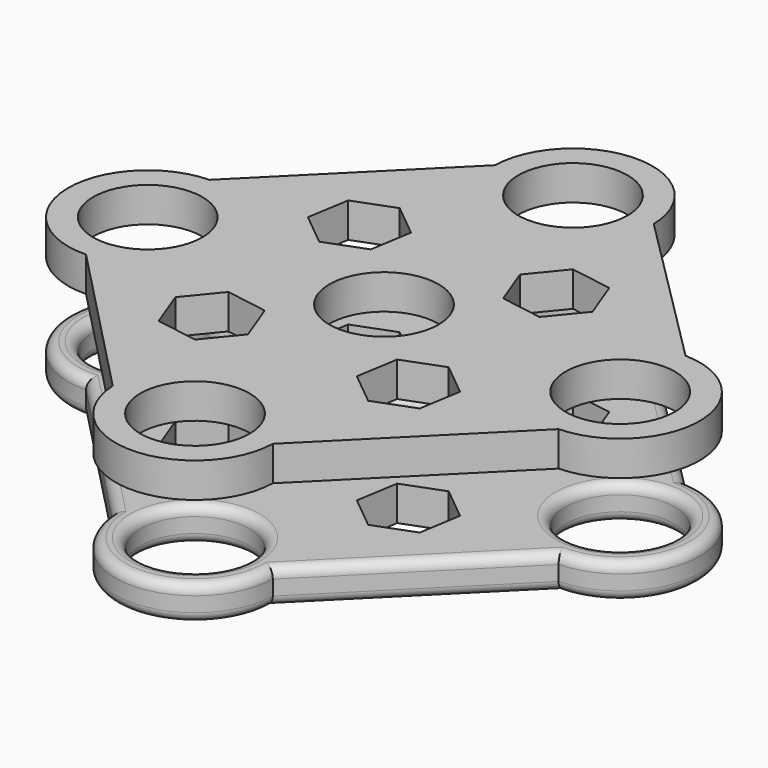
from build123d import *

# Parameters (mm, degrees)
F0_R     = 11
F1_DEPTH = 7
F3_R     = 2
F4_R     = 1.99999


# Not quite as in the source:
# - a fillet or chamfer is up to 0.001 mm smaller than in the source, because OpenCascade refuses the exact size


with BuildPart() as f1:
    # F0 (on Top) → F1 (new body)
    with BuildSketch(Plane.XY):
        with BuildLine():
            Line((-15.9957736565, 47.9499164564), (-47.9659518715, 15.9953969734))
            ThreePointArc((-47.9659518715, 15.9953969734), (-63.5777739911, -0.3757513624), (-47.2144492409, -15.9957734767))
            Line((-47.2144492409, -15.9957734767), (-15.9838429391, -48.3010503735))
            ThreePointArc((-15.9838429391, -48.3010503735), (0.1596400242, -63.5813903344), (15.9950047504, -47.9819654893))
            Line((15.9950047504, -47.9819654893), (47.9819799, -15.9950043902))
            ThreePointArc((47.9819799, -15.9950043902), (63.5821787222, 0.0160362946), (47.9499165377, 15.9957736546))
            Line((47.9499165377, 15.9957736546), (15.9961341611, 47.9338853509))
            ThreePointArc((15.9961341611, 47.9338853509), (0.0080175792, 63.5821847497), (-15.9957736565, 47.9499164564))
        make_face()
        with Locations((0, -47.5821867585)):
            Circle(F0_R, mode=Mode.SUBTRACT)
        with Locations((-47.5821867585, 0)):
            Circle(F0_R, mode=Mode.SUBTRACT)
        Polygon((-24.1507935557, -26.5329984332), (-27.1666148322, -18.5563192395), (-21.7665186508, -11.9562018039), (-13.350601193, -13.3327635621), (-10.3347799165, -21.3094427558), (-15.7348760979, -27.9095601914), align=None, mode=Mode.SUBTRACT)
        Circle(F0_R, mode=Mode.SUBTRACT)
        Polygon((27.9095601914, -15.7348760979), (26.5329984332, -24.1507935557), (18.5563192395, -27.1666148322), (11.9562018039, -21.7665186508), (13.3327635621, -13.350601193), (21.3094427558, -10.3347799165), align=None, mode=Mode.SUBTRACT)
        with Locations((47.5821867585, 0)):
            Circle(F0_R, mode=Mode.SUBTRACT)
        Polygon((-27.9095601914, 15.7348760979), (-26.5329984332, 24.1507935557), (-18.5563192395, 27.1666148322), (-11.9562018039, 21.7665186508), (-13.3327635621, 13.350601193), (-21.3094427558, 10.3347799165), align=None, mode=Mode.SUBTRACT)
        with Locations((0, 47.5821867585)):
            Circle(F0_R, mode=Mode.SUBTRACT)
        Polygon((15.7348760979, 27.9095601914), (24.1507935557, 26.5329984332), (27.1666148322, 18.5563192395), (21.7665186508, 11.9562018039), (13.350601193, 13.3327635621), (10.3347799165, 21.3094427558), align=None, mode=Mode.SUBTRACT)
    extrude(amount=F1_DEPTH)


with BuildPart() as f2_1:
    # F2: copy of F1
    add(f1.part.moved(Location((0, 0, 22))))


with BuildPart() as f1_1:
    add(f1.part)

    # F3
    f3_edges = [f1_1.edges().sort_by_distance(p)[0] for p in [
        (-31.980863, 31.972657, 7),
    ]]
    fillet(f3_edges, radius=F3_R)

    # F4 (radius 2 in the source; OpenCascade refuses exactly that, so slightly less here)
    f4_edges = [f1_1.edges().sort_by_distance(p)[0] for p in [
        (0.008018, 63.582185, 7),
        (31.973025, 31.96483, 7),
        (63.582179, 0.016036, 7),
        (31.988492, -31.988485, 7),
        (0.15964, -63.58139, 7),
        (-31.599146, -32.148412, 7),
        (-63.577774, -0.375751, 7),
        (-11, 0, 7),
        (-31.980863, 31.972657, 0),
        (0.008018, 63.582185, 0),
        (31.973025, 31.96483, 0),
        (63.582179, 0.016036, 0),
        (31.988492, -31.988485, 0),
        (0.15964, -63.58139, 0),
        (-31.599146, -32.148412, 0),
        (-63.577774, -0.375751, 0),
        (-11, 0, 0),
        (-11, 47.582187, 7),
        (36.582187, 0, 7),
        (-11, -47.582187, 7),
        (-58.582187, 0, 7),
        (-58.582187, 0, 0),
        (-11, 47.582187, 0),
        (36.582187, 0, 0),
        (-11, -47.582187, 0),
    ]]
    fillet(f4_edges, radius=F4_R)


solid = Compound([f2_1.part, f1_1.part])
